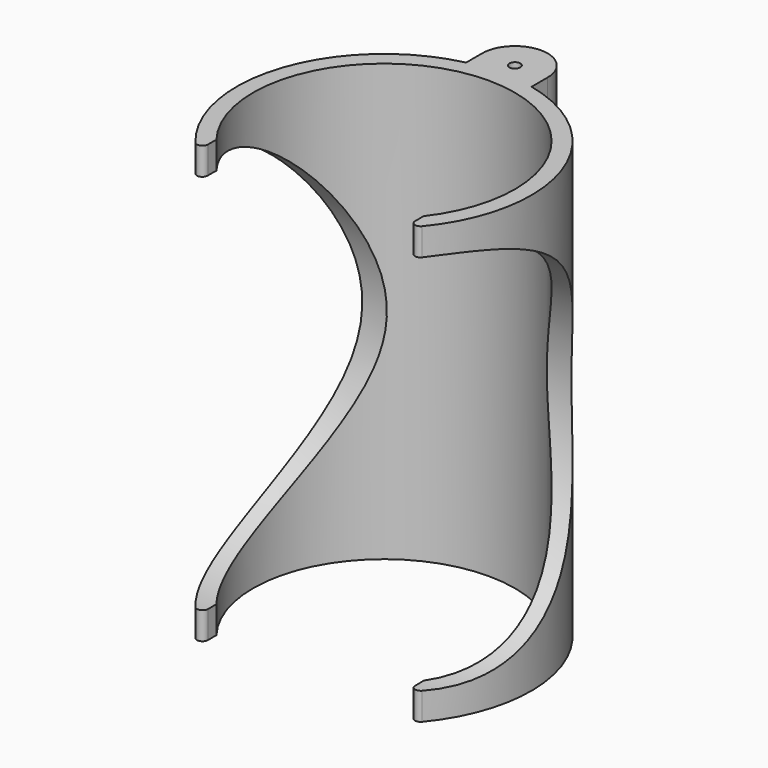
from build123d import *

# Parameters (mm, degrees)
F1_DEPTH    = 40
F2_R        = 17.5
F3_DEPTH    = 15
F5_R        = 0.5
F6_DEPTH    = 40
F7_T1_DEPTH = 9.1201245228
F7_T3_DEPTH = 9.1201245228


# Not quite as in the source:
# - a fillet or chamfer that OpenCascade refuses, or shapes differently, is made with other operations: its cross-section is extruded or revolved along the edge and cut away or added


with BuildPart() as f1:
    # F0 (on Top) → F1 (new body)
    with BuildSketch(Plane.XY):
        with BuildLine():
            ThreePointArc((-9.5, -7.3314391493), (0, 12), (9.5, -7.3314391493))
            Line((9.5, -7.3314391493), (9.5, -9.5916630466))
            ThreePointArc((9.5, -9.5916630466), (0, 13.5), (-9.5, -9.5916630466))
            Line((-9.5, -9.5916630466), (-9.5, -7.3314391493))
        make_face()
    extrude(amount=F1_DEPTH)


with BuildPart() as f3:
    # F2 (on Right) → F3 (new body, symmetric)
    with BuildSketch(Plane.YZ):
        with Locations((-8, 20)):
            Circle(F2_R)
    extrude(amount=F3_DEPTH, both=True)


with BuildPart() as f1_1:
    add(f1.part)

    # F4: cut F3
    add(f3.part, mode=Mode.SUBTRACT)

    # F5 (on Top) → F6 (join)
    with BuildSketch(Plane.XY):
        with BuildLine():
            Line((2.9997656158, 13.1625), (2.9997656158, 14.9625))
            ThreePointArc((2.9997656158, 14.9625), (0, 18), (-2.9997656158, 14.9625))
            Line((-2.9997656158, 14.9625), (-2.9997656158, 13.1625))
            ThreePointArc((-2.9997656158, 13.1625), (0, 13.5), (2.9997656158, 13.1625))
        make_face()
        with Locations((0, 15)):
            Circle(F5_R, mode=Mode.SUBTRACT)
    extrude(amount=F6_DEPTH)

    # F7: fillet of radius 0.5 on 4 edges, made by hand

    # F7_s2 → F7_t1 (cut)
    with BuildSketch(Plane.XY.offset(34.1536712775)):
        with BuildLine():
            ThreePointArc((-10.3846153846, -8.6261093961), (-9.8301584449, -8.7768938345), (-9.5, -8.3066238629))
            Line((-9.5, -8.3066238629), (-9.5, -9.5916630466))
            ThreePointArc((-9.5, -9.5916630466), (-9.9540220872, -9.1196186482), (-10.3846153846, -8.6261093961))
        make_face()
        with BuildLine():
            ThreePointArc((10.3846153846, -8.6261093961), (9.8301584449, -8.7768938345), (9.5, -8.3066238629))
            Line((9.5, -8.3066238629), (9.5, -9.5916630466))
            ThreePointArc((9.5, -9.5916630466), (9.9540220872, -9.1196186482), (10.3846153846, -8.6261093961))
        make_face()
    extrude(amount=F7_T1_DEPTH, mode=Mode.SUBTRACT)

    # F7_s4 → F7_t3 (cut)
    with BuildSketch(Plane.XY.offset(-3.2737958003)):
        with BuildLine():
            ThreePointArc((9.5, -8.3066238629), (9.8301584449, -8.7768938345), (10.3846153846, -8.6261093961))
            ThreePointArc((10.3846153846, -8.6261093961), (9.9540220872, -9.1196186482), (9.5, -9.5916630466))
            Line((9.5, -9.5916630466), (9.5, -8.3066238629))
        make_face()
        with BuildLine():
            ThreePointArc((-9.5, -8.3066238629), (-9.8301584449, -8.7768938345), (-10.3846153846, -8.6261093961))
            ThreePointArc((-10.3846153846, -8.6261093961), (-9.9540220872, -9.1196186482), (-9.5, -9.5916630466))
            Line((-9.5, -9.5916630466), (-9.5, -8.3066238629))
        make_face()
    extrude(amount=F7_T3_DEPTH, mode=Mode.SUBTRACT)


solid = f1_1.part
